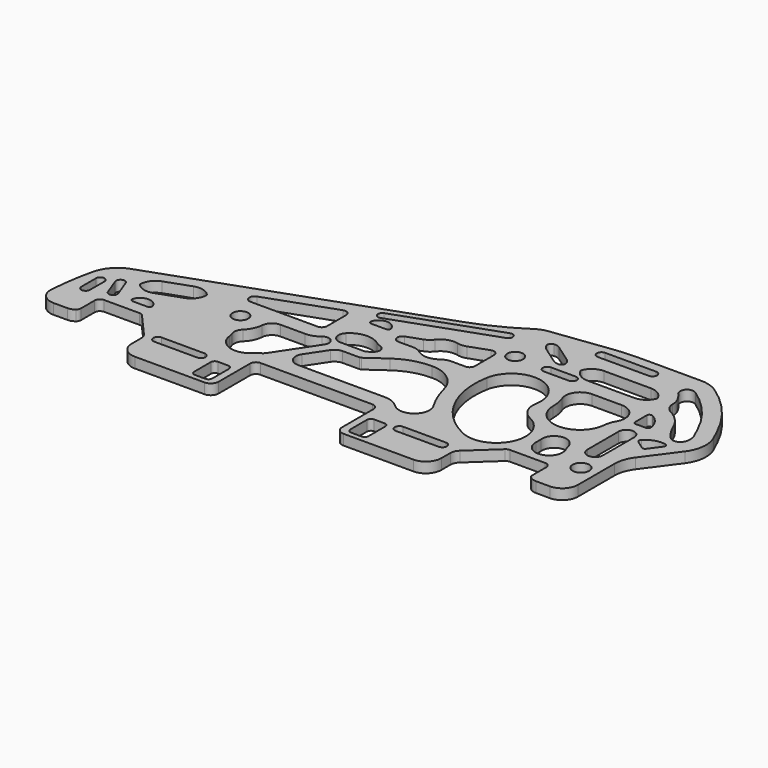
from build123d import *

# Parameters (mm, degrees)
F0_R     = 1.5
F0_R_2   = 1.6
F1_DEPTH = 2


# Not quite as in the source:
# - ends of sketch curves that miss each other by under 0.0002 mm in the source are joined


with BuildPart() as f1:
    # F0 (on Top) → F1 (new body)
    with BuildSketch(Plane.XY):
        with BuildLine():
            Line((40.512603, 23.481789), (29.131138, 23.481789))
            ThreePointArc((29.131138, 23.481789), (26.3012013624, 23.3918093627), (23.4826970067, 23.1222339475))
            Line((23.4826970067, 23.1222339475), (12.541684, 21.723653))
            ThreePointArc((12.541684, 21.723653), (11.4330843738, 21.4505213213), (10.4153498294, 20.9330172577))
            ThreePointArc((10.4153498294, 20.9330172577), (5.7781088608, 18.252530295), (0.8502767914, 16.153605586))
            Line((0.8502767914, 16.153605586), (-49.030999, -1.599885))
            ThreePointArc((-49.030999, -1.599885), (-51.4858947597, -3.2465284629), (-52.8566147278, -5.8655120647))
            ThreePointArc((-52.8566147278, -5.8655120647), (-53.6653577915, -10.0516677643), (-54.1163267723, -14.2913130145))
            ThreePointArc((-54.1163267723, -14.2913130145), (-53.3100074829, -16.5346616205), (-51.12238, -17.481789))
            Line((-51.12238, -17.481789), (-48.440844, -17.481789))
            ThreePointArc((-48.440844, -17.481789), (-47.7835331419, -17.3706887951), (-47.1992496549, -17.0497314358))
            ThreePointArc((-47.1992496549, -17.0497314358), (-46.9198255904, -16.7011924445), (-46.820047, -16.26576))
            Line((-46.820047, -16.26576), (-46.820047, -12.981789))
            ThreePointArc((-46.820047, -12.981789), (-46.5271537812, -12.2746822188), (-45.820047, -11.981789))
            Line((-45.820047, -11.981789), (-39.020047, -11.981789))
            ThreePointArc((-39.020047, -11.981789), (-38.5805485029, -12.0835456749), (-38.2304938172, -12.3681068579))
            Line((-38.2304938172, -12.3681068579), (-34.218141, -16.914727))
            ThreePointArc((-34.218141, -16.914727), (-33.8469994743, -17.5306782331), (-33.717714, -18.238087))
            Line((-33.717714, -18.238087), (-33.717714, -20.481789))
            ThreePointArc((-33.717714, -20.481789), (-32.8390343436, -22.6031093436), (-30.717714, -23.481789))
            Line((-30.717714, -23.481789), (-17.317714, -23.481789))
            ThreePointArc((-17.317714, -23.481789), (-16.2570538282, -23.0424491718), (-15.817714, -21.981789))
            Line((-15.817714, -21.981789), (-15.817714, -14.406789))
            ThreePointArc((-15.817714, -14.406789), (-15.4955314593, -13.6289715407), (-14.717714, -13.306789))
            Line((-14.717714, -13.306789), (6.782286, -13.306789))
            ThreePointArc((6.782286, -13.306789), (7.5601034593, -13.6289715407), (7.882286, -14.406789))
            Line((7.882286, -14.406789), (7.882286, -21.981789))
            ThreePointArc((7.882286, -21.981789), (8.3216258282, -23.0424491718), (9.382286, -23.481789))
            Line((9.382286, -23.481789), (22.782286, -23.481789))
            ThreePointArc((22.782286, -23.481789), (24.9036063436, -22.6031093436), (25.782286, -20.481789))
            Line((25.782286, -20.481789), (25.782286, -18.355608))
            ThreePointArc((25.782286, -18.355608), (25.9495741205, -17.554878853), (26.4234531668, -16.8881021801))
            Line((26.4234531668, -16.8881021801), (31.405835, -12.274682))
            ThreePointArc((31.405835, -12.274682), (31.7302578943, -12.0579093322), (32.112941, -11.981789))
            Line((32.112941, -11.981789), (38.912941, -11.981789))
            ThreePointArc((38.912941, -11.981789), (39.6200477812, -12.2746822188), (39.912941, -12.981789))
            Line((39.912941, -12.981789), (39.912941, -16.653547))
            ThreePointArc((39.912941, -16.653547), (40.6236607426, -17.2627318866), (41.533739, -17.481789))
            Line((41.533739, -17.481789), (44.195651, -17.481789))
            ThreePointArc((44.195651, -17.481789), (46.3169713436, -16.6031093436), (47.195651, -14.481789))
            Line((47.195651, -14.481789), (47.195651, -5.721688))
            ThreePointArc((47.195651, -5.721688), (47.4967831217, -3.8447476959), (48.3699526351, -2.1562097304))
            Line((48.3699526351, -2.1562097304), (52.948078, 4.040056))
            ThreePointArc((52.948078, 4.040056), (54.0924061177, 7.0065457232), (53.5602269903, 10.1412439955))
            Line((53.5602269903, 10.1412439955), (52.595339, 12.210453))
            ThreePointArc((52.595339, 12.210453), (48.9319736591, 17.9164640466), (43.8846811941, 22.4445592857))
            ThreePointArc((43.8846811941, 22.4445592857), (42.2766010714, 23.2166221104), (40.512603, 23.481789))
        make_face()
        with BuildLine():
            ThreePointArc((-31.467714, -17.856789), (-32.342714, -16.981789), (-31.467714, -16.106789))
            Line((-31.467714, -16.106789), (-23.217714, -16.106789))
            ThreePointArc((-23.217714, -16.106789), (-22.342714, -16.981789), (-23.217714, -17.856789))
            Line((-23.217714, -17.856789), (-31.467714, -17.856789))
        make_face(mode=Mode.SUBTRACT)
        with BuildLine():
            Line((-17.967714, -22.481789), (-19.967714, -22.481789))
            ThreePointArc((-19.967714, -22.481789), (-20.4980440859, -22.2621190859), (-20.717714, -21.731789))
            Line((-20.717714, -21.731789), (-20.717714, -17.731789))
            ThreePointArc((-20.717714, -17.731789), (-20.4980440859, -17.2014589141), (-19.967714, -16.981789))
            Line((-19.967714, -16.981789), (-17.967714, -16.981789))
            ThreePointArc((-17.967714, -16.981789), (-17.4373839141, -17.2014589141), (-17.217714, -17.731789))
            Line((-17.217714, -17.731789), (-17.217714, -21.731789))
            ThreePointArc((-17.217714, -21.731789), (-17.4373839141, -22.2621190859), (-17.967714, -22.481789))
        make_face(mode=Mode.SUBTRACT)
        with BuildLine():
            ThreePointArc((-49.5275950002, -10.739971), (-50.352612, -11.5649539998), (-51.1775949998, -10.739937))
            Line((-51.177595, -10.739937), (-51.177524, -7.239937))
            ThreePointArc((-51.1775239998, -7.239937), (-50.352507, -6.4149540002), (-49.5275240002, -7.239971))
            Line((-49.527524, -7.239971), (-49.527595, -10.739971))
        make_face(mode=Mode.SUBTRACT)
        with BuildLine():
            ThreePointArc((-45.4957372463, -8.9390500929), (-45.9766256551, -10.0020625887), (-47.0396384236, -9.5211747827))
            Line((-47.0396384236, -9.5211747827), (-48.274448, -6.246232))
            ThreePointArc((-48.274448, -6.246232), (-47.7935590722, -5.1832193085), (-46.7305463707, -5.6641077627))
            Line((-46.7305463707, -5.6641077627), (-45.4957372463, -8.9390500929))
        make_face(mode=Mode.SUBTRACT)
        with BuildLine():
            ThreePointArc((-42.6629909692, -8.9668840109), (-40.777373, -7.633551), (-38.8917550308, -8.9668840109))
            ThreePointArc((-38.8917550308, -8.9668840109), (-38.9549116649, -9.4222260715), (-39.36316, -9.633551))
            Line((-39.36316, -9.633551), (-42.191587, -9.633551))
            ThreePointArc((-42.191587, -9.633551), (-42.5998354313, -9.4222259354), (-42.6629909692, -8.9668840109))
        make_face(mode=Mode.SUBTRACT)
        with BuildLine():
            ThreePointArc((-34.9182417778, -0.9247827916), (-34.8118579238, -1.0992106617), (-34.7841268371, -1.3016300114))
            ThreePointArc((-34.7841268371, -1.3016300114), (-35.3872435627, -2.9067375552), (-36.7710009647, -3.9193260992))
            Line((-36.7710009647, -3.9193260992), (-41.481581, -5.595761))
            ThreePointArc((-41.481581, -5.595761), (-43.1939324368, -5.6850383639), (-44.6754877704, -4.8218397847))
            ThreePointArc((-44.6754877704, -4.8218397847), (-44.7818720762, -4.6474123383), (-44.8096031629, -4.4449929886))
            ThreePointArc((-44.8096031629, -4.4449929886), (-44.2064864373, -2.8398854448), (-42.8227290353, -1.8272969008))
            Line((-42.8227290353, -1.8272969008), (-38.112149, -0.150862))
            ThreePointArc((-38.112149, -0.150862), (-36.3997975632, -0.0615846361), (-34.9182417778, -0.9247827916))
        make_face(mode=Mode.SUBTRACT)
        with BuildLine():
            ThreePointArc((-12.8914672348, -0.8369777084), (-11.1748635352, -0.8897115606), (-10.9642623193, -2.5941634515))
            Line((-10.9642623193, -2.5941634515), (-15.985232, -10.164331))
            ThreePointArc((-15.985232, -10.164331), (-16.2982295126, -10.5310910952), (-16.68990598, -10.8122850364))
            ThreePointArc((-16.68990598, -10.8122850364), (-17.178069055, -11.1270553213), (-17.6168518029, -11.5076511971))
            ThreePointArc((-17.6168518029, -11.5076511971), (-21.3317967336, -12.3891200944), (-23.788276857, -9.4661921264))
            add(Edge.make_bspline(
                [(-24.018798, -8.541721), (-23.914252, -8.835884), (-23.835359, -9.147054), (-23.788276857, -9.4661921264)],
                knots=[0, 0, 0, 0, 1, 1, 1, 1], degree=3))
            ThreePointArc((-24.018798, -8.541721), (-24.0818260098, -7.4169212268), (-23.5269228293, -6.4364981759))
            ThreePointArc((-23.5269228293, -6.4364981759), (-22.5887878527, -5.1230141758), (-22.1744970765, -3.5629819939))
            ThreePointArc((-22.1744970765, -3.5629819939), (-21.5378523692, -2.2521936612), (-20.180775, -1.721323))
            Line((-20.180775, -1.721323), (-15.399992, -1.721323))
            ThreePointArc((-15.399992, -1.721323), (-14.0700706748, -1.4937637575), (-12.8914672348, -0.8369777084))
        make_face(mode=Mode.SUBTRACT)
        with Locations((-26.660371, -3.206714)):
            Circle(F0_R, mode=Mode.SUBTRACT)
        with BuildLine():
            Line((12.032286, -22.481789), (10.032286, -22.481789))
            ThreePointArc((10.032286, -22.481789), (9.5019559141, -22.2621190859), (9.282286, -21.731789))
            Line((9.282286, -21.731789), (9.282286, -17.731789))
            ThreePointArc((9.282286, -17.731789), (9.5019559141, -17.2014589141), (10.032286, -16.981789))
            Line((10.032286, -16.981789), (12.032286, -16.981789))
            ThreePointArc((12.032286, -16.981789), (12.5626160859, -17.2014589141), (12.782286, -17.731789))
            Line((12.782286, -17.731789), (12.782286, -21.731789))
            ThreePointArc((12.782286, -21.731789), (12.5626160859, -22.2621190859), (12.032286, -22.481789))
        make_face(mode=Mode.SUBTRACT)
        with BuildLine():
            ThreePointArc((14.907286, -17.856789), (14.032286, -16.981789), (14.907286, -16.106789))
            Line((14.907286, -16.106789), (23.157286, -16.106789))
            ThreePointArc((23.157286, -16.106789), (24.032286, -16.981789), (23.157286, -17.856789))
            Line((23.157286, -17.856789), (14.907286, -17.856789))
        make_face(mode=Mode.SUBTRACT)
        with BuildLine():
            ThreePointArc((-0.4859768424, -0.0560492228), (2.5782626644, 1.4685681541), (5.960388, 1.993211))
            ThreePointArc((5.960388, 1.993211), (9.8546582158, 0.6492086336), (12.0910173552, -2.8106151588))
            ThreePointArc((12.0910173552, -2.8106151588), (12.9614193732, -5.4513852217), (14.2260258996, -7.9276800614))
            ThreePointArc((14.2260258996, -7.9276800614), (13.5437578661, -11.7361360382), (9.6814241094, -11.5076508906))
            ThreePointArc((9.6814241094, -11.5076508906), (8.3512880727, -10.6188829167), (6.782286, -10.306789))
            Line((6.782286, -10.306789), (-9.953353, -10.306789))
            ThreePointArc((-9.953353, -10.306789), (-11.7155854955, -9.252588467), (-11.620071555, -7.2013256319))
            Line((-11.620071555, -7.2013256319), (-9.157645, -3.4887))
            ThreePointArc((-9.157645, -3.4887), (-8.436726467, -2.8319305045), (-7.490927, -2.594163))
            Line((-7.490927, -2.594163), (-4.233575, -2.594163))
            ThreePointArc((-4.233575, -2.594163), (-4.0820979302, -2.570665568), (-3.944858149, -2.5023817893))
            Line((-3.944858149, -2.5023817893), (-0.4859768424, -0.0560492228))
        make_face(mode=Mode.SUBTRACT)
        with BuildLine():
            ThreePointArc((23.2842162035, -12.1670365636), (16.2718885147, -5.4541932436), (14.7951548491, 4.1402980266))
            ThreePointArc((14.7951548491, 4.1402980266), (21.2825074947, 8.6827924698), (25.8250013994, 2.1954391059))
            ThreePointArc((25.8250013994, 2.1954391059), (26.2064097269, -0.2826085461), (28.0175408191, -2.016389388))
            ThreePointArc((28.0175408191, -2.016389388), (30.7262015878, -9.4583753078), (23.2842162035, -12.1670365636))
        make_face(mode=Mode.SUBTRACT)
        with BuildLine():
            ThreePointArc((33.6179031498, -6.3682089864), (35.5921266207, -3.8339317975), (38.2510782143, -5.6367339515))
            ThreePointArc((38.2510782143, -5.6367339515), (38.3885509252, -6.1180286043), (38.5786257021, -6.5810781421))
            ThreePointArc((38.5786257021, -6.5810781421), (36.7333598567, -10.2510263374), (33.6375186543, -7.5511569801))
            ThreePointArc((33.6375186543, -7.5511569801), (33.6496094194, -6.95931986), (33.6179031498, -6.3682089864))
        make_face(mode=Mode.SUBTRACT)
        with Locations((44.077012, -9.856887)):
            Circle(F0_R_2, mode=Mode.SUBTRACT)
        with BuildLine():
            Line((41.14007, -4.643381), (41.14007, 2.856619))
            ThreePointArc((41.14007, 2.856619), (42.64007, 4.356619), (44.14007, 2.856619))
            Line((44.14007, 2.856619), (44.14007, -4.643381))
            ThreePointArc((44.14007, -4.643381), (42.64007, -6.143381), (41.14007, -4.643381))
        make_face(mode=Mode.SUBTRACT)
        with BuildLine():
            ThreePointArc((-14.399992, 2.278677), (-14.6928852188, 1.5715702188), (-15.399992, 1.278677))
            Line((-15.399992, 1.278677), (-28.302898, 1.278677))
            ThreePointArc((-28.302898, 1.278677), (-29.2883186889, 2.108541566), (-28.6382079531, 3.2207848682))
            Line((-28.6382079531, 3.2207848682), (-15.735302, 7.813122))
            ThreePointArc((-15.735302, 7.813122), (-14.8234982676, 7.6881155705), (-14.399992, 6.871014))
            Line((-14.399992, 6.871014), (-14.399992, 2.278677))
        make_face(mode=Mode.SUBTRACT)
        with BuildLine():
            ThreePointArc((-10.7614838372, 2.2449998422), (-8.073944308, 3.5275248105), (-5.201188416, 2.7432974202))
            ThreePointArc((-5.201188416, 2.7432974202), (-4.6693203129, 2.4211658961), (-4.0939581553, 2.1853465171))
            ThreePointArc((-4.0939581553, 2.1853465171), (-3.2783121553, 1.2285041707), (-3.7696761681, 0.0711852377))
            Line((-3.7696761681, 0.0711852377), (-4.580646, -0.502382))
            ThreePointArc((-4.580646, -0.502382), (-4.7178859302, -0.570665568), (-4.869363, -0.594163))
            Line((-4.869363, -0.594163), (-9.559223, -0.594163))
            ThreePointArc((-9.559223, -0.594163), (-11.1008358519, 0.427164926), (-10.7614838372, 2.2449998422))
        make_face(mode=Mode.SUBTRACT)
        with BuildLine():
            ThreePointArc((-6.4102286418, 7.7020681266), (-6.4733845687, 7.2467260646), (-6.881633, 7.035401))
            Line((-6.881633, 7.035401), (-9.71006, 7.035401))
            ThreePointArc((-9.71006, 7.035401), (-10.1183083351, 7.2467259285), (-10.1814644693, 7.7020678124))
            ThreePointArc((-10.1814644693, 7.7020678124), (-8.295847, 9.035401), (-6.4102286418, 7.7020681266))
        make_face(mode=Mode.SUBTRACT)
        with BuildLine():
            Line((9.03337, 16.067494), (-9.808786, 9.36129))
            ThreePointArc((-9.808786, 9.36129), (-10.8626559011, 9.8618980352), (-10.3620479648, 10.9157679011))
            Line((-10.3620479648, 10.9157679011), (8.480108, 17.621972))
            ThreePointArc((8.480108, 17.621972), (9.5339779011, 17.1213639648), (9.03337, 16.067494))
        make_face(mode=Mode.SUBTRACT)
        with BuildLine():
            Line((10.033684, 4.993211), (7.33223, 4.993211))
            ThreePointArc((7.33223, 4.993211), (6.3835467019, 4.8392608942), (5.53223, 4.393211))
            ThreePointArc((5.53223, 4.393211), (3.58223, 3.743211), (1.63223, 4.393211))
            ThreePointArc((1.63223, 4.393211), (0.7809132981, 4.8392608942), (-0.16777, 4.993211))
            Line((-0.16777, 4.993211), (-2.869223, 4.993211))
            ThreePointArc((-2.869223, 4.993211), (-3.8546436889, 5.823075566), (-3.2045329531, 6.9353188682))
            Line((-3.2045329531, 6.9353188682), (-0.399099, 7.933815))
            ThreePointArc((-0.399099, 7.933815), (0.3694752692, 8.3412268711), (0.9888548126, 8.9520131415))
            ThreePointArc((0.9888548126, 8.9520131415), (2.4924719179, 10.0550613103), (4.354879037, 10.150031151))
            ThreePointArc((4.354879037, 10.150031151), (5.2208742596, 10.067911827), (6.0740241752, 10.2376955078))
            Line((6.0740241752, 10.2376955078), (9.698373, 11.527656))
            ThreePointArc((9.698373, 11.527656), (10.6101773475, 11.4026498421), (11.033684, 10.585548))
            Line((11.033684, 10.585548), (11.033684, 5.993211))
            ThreePointArc((11.033684, 5.993211), (10.7407907812, 5.2861042188), (10.033684, 4.993211))
        make_face(mode=Mode.SUBTRACT)
        with BuildLine():
            ThreePointArc((27.7891688027, 6.0074479251), (28.1067686801, 8.6291374327), (30.445019, 9.856619))
            Line((30.445019, 9.856619), (36.14007, 9.856619))
            ThreePointArc((36.14007, 9.856619), (38.8274592707, 8.2886229698), (38.7847711817, 5.1775378906))
            ThreePointArc((38.7847711817, 5.1775378906), (38.3536542424, 4.2265187664), (38.15332528, 3.2017419785))
            ThreePointArc((38.15332528, 3.2017419785), (35.2828977993, -0.9670181189), (30.2396183016, -0.5389475693))
            ThreePointArc((30.2396183016, -0.5389475693), (28.821344139, 1.0783944365), (28.310078, 3.167869))
            ThreePointArc((28.310078, 3.167869), (28.1787730258, 4.6113504133), (27.7891688027, 6.0074479251))
        make_face(mode=Mode.SUBTRACT)
        with BuildLine():
            ThreePointArc((45.4988994737, 2.8491105135), (47.1838928944, 3.898776074), (49.1633500895, 4.0496065395))
            ThreePointArc((49.1633500895, 4.0496065395), (49.5448804105, 3.7441256856), (49.4836143222, 3.2592237619))
            Line((49.4836143222, 3.2592237619), (47.839895, 1.034619))
            ThreePointArc((47.839895, 1.034619), (47.5120091165, 0.8372928137), (47.1406281151, 0.9296131558))
            Line((47.1406281151, 0.9296131558), (45.559631, 2.097782))
            ThreePointArc((45.559631, 2.097782), (45.358387471, 2.4596336496), (45.4988994737, 2.8491105135))
        make_face(mode=Mode.SUBTRACT)
        with BuildLine():
            Line((43.605819, 6.356619), (41.64007, 6.356619))
            ThreePointArc((41.64007, 6.356619), (41.2865166094, 6.5030656094), (41.14007, 6.856619))
            Line((41.14007, 6.856619), (41.14007, 9.622605))
            ThreePointArc((41.14007, 9.622605), (41.3789535753, 10.049006469), (41.8673428511, 10.0679667082))
            ThreePointArc((41.8673428511, 10.0679667082), (43.3697322766, 8.7703439483), (44.1011495134, 6.9248010707))
            ThreePointArc((44.1011495134, 6.9248010707), (43.9827082142, 6.528054668), (43.605819, 6.356619))
        make_face(mode=Mode.SUBTRACT)
        with Locations((13.783684, 12.215472)):
            Circle(F0_R, mode=Mode.SUBTRACT)
        with BuildLine():
            ThreePointArc((24.980271, 12.789048), (25.830271, 11.939048), (24.980271, 11.089048))
            Line((24.980271, 11.089048), (20.180271, 11.089048))
            ThreePointArc((20.180271, 11.089048), (19.330271, 11.939048), (20.180271, 12.789048))
            Line((20.180271, 12.789048), (24.980271, 12.789048))
        make_face(mode=Mode.SUBTRACT)
        with BuildLine():
            ThreePointArc((20.3844069997, 16.3123449996), (20.8498540778, 15.8570545203), (21.1443936056, 15.2763851913))
            ThreePointArc((21.1443936056, 15.2763851913), (21.0449245196, 14.6290714469), (20.470669016, 14.3142066285))
            ThreePointArc((20.470669016, 14.3142066285), (19.8242796139, 14.3923821589), (19.2372540003, 14.6740410004))
            Line((19.2372540003, 14.6740410004), (15.960646, 16.968347))
            ThreePointArc((15.960646, 16.968347), (15.4951981645, 17.4236371495), (15.2006583944, 18.0043068087))
            ThreePointArc((15.2006583944, 18.0043068087), (15.3001272069, 18.6516211625), (15.874382984, 18.9664863715))
            ThreePointArc((15.874382984, 18.9664863715), (16.5207725341, 18.8883100897), (17.1077983287, 18.6066514695))
            Line((17.1077983287, 18.6066514695), (20.3844069997, 16.3123449996))
        make_face(mode=Mode.SUBTRACT)
        with BuildLine():
            Line((36.14007, 12.856619), (27.14007, 12.856619))
            ThreePointArc((27.14007, 12.856619), (25.4969023973, 13.3466388747), (24.3905246497, 14.6566188471))
            ThreePointArc((24.3905246497, 14.6566188471), (24.348782, 14.856619), (24.3905245216, 15.0566192088))
            ThreePointArc((24.3905245216, 15.0566192088), (25.4969023973, 16.3665991253), (27.14007, 16.856619))
            Line((27.14007, 16.856619), (36.14007, 16.856619))
            ThreePointArc((36.14007, 16.856619), (37.7832377701, 16.3665990157), (38.8896155103, 15.0566187863))
            ThreePointArc((38.8896155103, 15.0566187863), (38.931358, 14.856619), (38.8896156384, 14.6566191578))
            ThreePointArc((38.8896156384, 14.6566191578), (37.7832377701, 13.3466389843), (36.14007, 12.856619))
        make_face(mode=Mode.SUBTRACT)
        with BuildLine():
            ThreePointArc((42.198642103, 19.9631741516), (46.6474415377, 15.9720070566), (49.876415804, 10.9425979086))
            Line((49.876415804, 10.9425979086), (50.841303, 8.873389))
            ThreePointArc((50.841303, 8.873389), (51.1184389035, 7.7592589312), (50.9567879312, 6.6226150239))
            ThreePointArc((50.9567879312, 6.6226150239), (49.8994761378, 5.6868299941), (48.5507912462, 6.104743233))
            ThreePointArc((48.5507912462, 6.104743233), (47.4304588961, 7.5260418462), (46.583603485, 9.1254387843))
            ThreePointArc((46.583603485, 9.1254387843), (45.2279031957, 11.2301550972), (43.2309791961, 12.7401383844))
            ThreePointArc((43.2309791961, 12.7401383844), (42.2826874722, 13.6171191134), (41.9313571569, 14.8600670011))
            ThreePointArc((41.9313571569, 14.8600670011), (41.8571774503, 15.5733902983), (41.6391609886, 16.256618995))
            ThreePointArc((41.6391609886, 16.256618995), (41.1458746049, 17.1644763515), (40.5041472747, 17.9742432592))
            ThreePointArc((40.5041472747, 17.9742432592), (40.4596542248, 19.7284379453), (42.198642103, 19.9631741516))
        make_face(mode=Mode.SUBTRACT)
        with BuildLine():
            Line((33.382697, 19.821789), (23.582697, 19.821789))
            ThreePointArc((23.582697, 19.821789), (22.707697, 20.696789), (23.582697, 21.571789))
            Line((23.582697, 21.571789), (33.382697, 21.571789))
            ThreePointArc((33.382697, 21.571789), (34.257697, 20.696789), (33.382697, 19.821789))
        make_face(mode=Mode.SUBTRACT)
    extrude(amount=F1_DEPTH)


solid = f1.part
